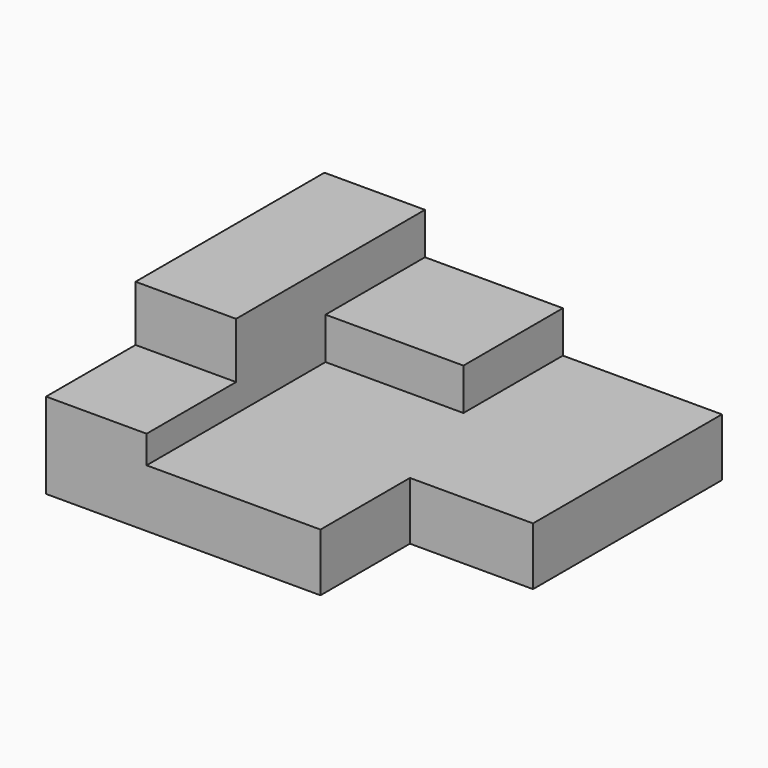
from build123d import *

# Parameters (mm, degrees)
F0_W      = 22.86
F0_H      = 10.16
F1_DEPTH  = 25
F2_W      = 7.1686236836
F2_H      = 5.1849592477
F3_DEPTH  = 5
F4_W      = 9.9097841885
F4_H      = 8.9319869876
F5_DEPTH  = 3
F6_W      = 10.2559335064
F6_H      = 16.0680130124
F7_DEPTH  = 6
F8_W      = 3.1437913674
F8_H      = 8.0340065062
F9_DEPTH  = 25
F10_W     = 8.0340065062
F10_H     = 6
F11_DEPTH = 7.2244124593
F12_W     = 7.2234124593
F12_H     = 8.0340065062
F13_DEPTH = 2
F14_DEPTH = 5.7


# Not quite as in the source:
# - a feature names something its author has since deleted; it is built from what else it names


with BuildPart() as f1:
    # F0 (on Front) → F1 (new body)
    with BuildSketch(Plane.XZ):
        with Locations((0.6582729786, 5.08)):
            Rectangle(F0_W, F0_H)
    extrude(amount=F1_DEPTH)

    # F2 (on face) → F3 (cut)
    with BuildSketch(Plane.XY.offset(10.16)):
        with Locations((-7.1874151796, -22.4075203761)):
            Rectangle(F2_W, F2_H)
    extrude(amount=-F3_DEPTH, mode=Mode.SUBTRACT)

    # F4 (on face) → F5 (cut)
    with BuildSketch(Plane.XY.offset(10.16)):
        with Locations((1.4065775322, -4.4659934938)):
            Rectangle(F4_W, F4_H)
    extrude(amount=-F5_DEPTH, mode=Mode.SUBTRACT)

    # F6 (on face) → F7 (cut)
    with BuildSketch(Plane.XY.offset(10.16)):
        with Locations((1.5796521911, -16.9659934938)):
            Rectangle(F6_W, F6_H)
        Polygon((6.3614696264, 0), (6.3614696264, -8.9319869876), (6.7076189443, -8.9319869876), (6.7076189443, -25), (12.0882729786, -25), (12.0882729786, 0), align=None)
    extrude(amount=-F7_DEPTH, mode=Mode.SUBTRACT)

    # F8 (on face) → F9 (cut)
    with BuildSketch(Plane.XY.offset(4.16)):
        with Locations((10.5163772949, -20.9829967469)):
            Rectangle(F8_W, F8_H)
    extrude(amount=-F9_DEPTH, mode=Mode.SUBTRACT)

    # F10 (on face) → F11 (cut, through all)
    with BuildSketch(Plane.YZ.offset(-3.5483145621)):
        with Locations((-20.9829967469, 7.16)):
            Rectangle(F10_W, F10_H)
    extrude(amount=-F11_DEPTH, mode=Mode.SUBTRACT)

    # F12 (on face) → F13 (join)
    with BuildSketch(Plane.XY.offset(4.16)):
        with Locations((-7.1600207917, -20.9829967469)):
            Rectangle(F12_W, F12_H)
    extrude(amount=F13_DEPTH)

    # F14 (add): a face of the model
    f14_faces = [f1.faces().sort_by_distance(p)[0] for p in [
        (12.0882729786, -8.4829967469, 2.08),
    ]]
    extrude(f14_faces, amount=F14_DEPTH)


solid = f1.part
